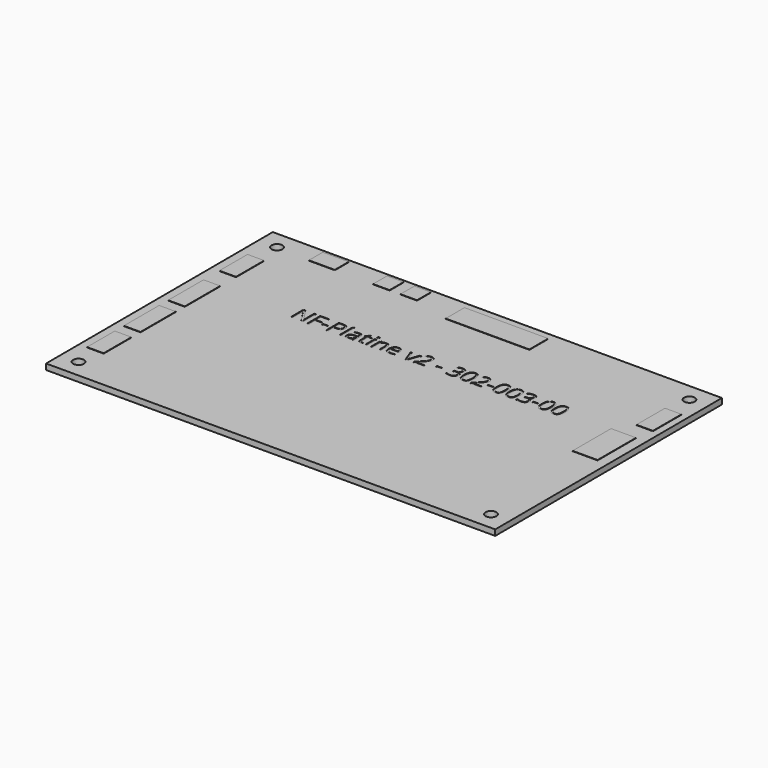
from build123d import *

# Parameters (mm, degrees)
F0_R         = 1.5
F0_W         = 4.612442106
F0_H         = 9.6228178591
F0_H_2       = 12.2249075212
F0_H_3       = 12.260917807
F0_H_4       = 9.7569040954
F0_W_2       = 7.1835308336
F0_H_5       = 4.8303045332
F0_W_3       = 4.5825974084
F0_W_4       = 6.908506155
F0_H_6       = 13.3309915545
F0_W_5       = 23.2019796968
F0_H_7       = 6.5229777246
F0_W_6       = 4.5825317502
F0_H_8       = 9.9142610561
F1_DEPTH     = 1.6
F2_TEXT_SIZE = 6.1743944469
F3_DEPTH     = 0.1
F4_DEPTH     = 0.1


# Not quite as in the source:
# - Text() gives the source's letters only with a copy of the font that has no kerning and outlines rounded to 1/6400 em; it was checked with that copy


with BuildPart() as f1:
    # F0 (on Top) → F1 (new body)
    with BuildSketch(Plane.XY):
        Polygon((-62.1453333333, -39.37), (62.3149554509, -39.37), (62.1453333333, 39.37), (-62.3149554509, 39.37), align=None)
        with Locations((-57.1453333333, -34.37)):
            Circle(F0_R, mode=Mode.SUBTRACT)
        with Locations((-57.6065722853, -23.1691235676)):
            Rectangle(F0_W, F0_H, mode=Mode.SUBTRACT)
        with Locations((-57.6065722853, -9.1032318305)):
            Rectangle(F0_W, F0_H_2, mode=Mode.SUBTRACT)
        with Locations((57.1453333333, -34.37)):
            Circle(F0_R, mode=Mode.SUBTRACT)
        with Locations((-57.6065722853, 6.2528505223)):
            Rectangle(F0_W, F0_H_3, mode=Mode.SUBTRACT)
        with Locations((-57.6065722853, 22.7434274275)):
            Rectangle(F0_W, F0_H_4, mode=Mode.SUBTRACT)
        with Locations((-57.1453333333, 34.37)):
            Circle(F0_R, mode=Mode.SUBTRACT)
        with Locations((-44.2407692317, 36.1824017018)):
            Rectangle(F0_W_2, F0_H_5, mode=Mode.SUBTRACT)
        with Locations((-27.747973334, 36.1824017018)):
            Rectangle(F0_W_3, F0_H_5, mode=Mode.SUBTRACT)
        with Locations((-20.1515958179, 36.1824017018)):
            Rectangle(F0_W_3, F0_H_5, mode=Mode.SUBTRACT)
        with Locations((55.9572540224, 6.365174806)):
            Rectangle(F0_W_4, F0_H_6, mode=Mode.SUBTRACT)
        with Locations((3.9263451472, 34.2132961377)):
            Rectangle(F0_W_5, F0_H_7, mode=Mode.SUBTRACT)
        with Locations((57.9382181168, 22.8221059078)):
            Rectangle(F0_W_6, F0_H_8, mode=Mode.SUBTRACT)
        with Locations((57.1453333333, 34.37)):
            Circle(F0_R, mode=Mode.SUBTRACT)
        with Locations((-57.6065722853, 22.7434274275)):
            Rectangle(F0_W, F0_H_4)
        with Locations((-57.6065722853, 6.2528505223)):
            Rectangle(F0_W, F0_H_3)
        with Locations((-57.6065722853, -9.1032318305)):
            Rectangle(F0_W, F0_H_2)
        with Locations((-57.6065722853, -23.1691235676)):
            Rectangle(F0_W, F0_H)
        with Locations((-44.2407692317, 36.1824017018)):
            Rectangle(F0_W_2, F0_H_5)
        with Locations((-27.747973334, 36.1824017018)):
            Rectangle(F0_W_3, F0_H_5)
        with Locations((-20.1515958179, 36.1824017018)):
            Rectangle(F0_W_3, F0_H_5)
        with Locations((3.9263451472, 34.2132961377)):
            Rectangle(F0_W_5, F0_H_7)
        with Locations((57.9382181168, 22.8221059078)):
            Rectangle(F0_W_6, F0_H_8)
        with Locations((55.9572540224, 6.365174806)):
            Rectangle(F0_W_4, F0_H_6)
    extrude(amount=-F1_DEPTH)

    # F2 (on face) → F3 (cut)
    with BuildSketch(Plane.XY):
        with Locations((-34.9935479462, 10.6949424371)):
            Text('NF-Platine v2 - 302-003-00', F2_TEXT_SIZE, font='Open Sans', text_align=(TextAlign.LEFT, TextAlign.BOTTOM))
    extrude(amount=-F3_DEPTH, mode=Mode.SUBTRACT)

    # F0 (on Top) → F4 (join)
    with BuildSketch(Plane.XY):
        with Locations((-57.6065722853, 22.7434274275)):
            Rectangle(F0_W, F0_H_4)
        with Locations((-57.6065722853, 6.2528505223)):
            Rectangle(F0_W, F0_H_3)
        with Locations((-57.6065722853, -9.1032318305)):
            Rectangle(F0_W, F0_H_2)
        with Locations((-57.6065722853, -23.1691235676)):
            Rectangle(F0_W, F0_H)
        with Locations((-44.2407692317, 36.1824017018)):
            Rectangle(F0_W_2, F0_H_5)
        with Locations((-27.747973334, 36.1824017018)):
            Rectangle(F0_W_3, F0_H_5)
        with Locations((-20.1515958179, 36.1824017018)):
            Rectangle(F0_W_3, F0_H_5)
        with Locations((3.9263451472, 34.2132961377)):
            Rectangle(F0_W_5, F0_H_7)
        with Locations((55.9572540224, 6.365174806)):
            Rectangle(F0_W_4, F0_H_6)
        with Locations((57.9382181168, 22.8221059078)):
            Rectangle(F0_W_6, F0_H_8)
    extrude(amount=F4_DEPTH)


solid = f1.part
